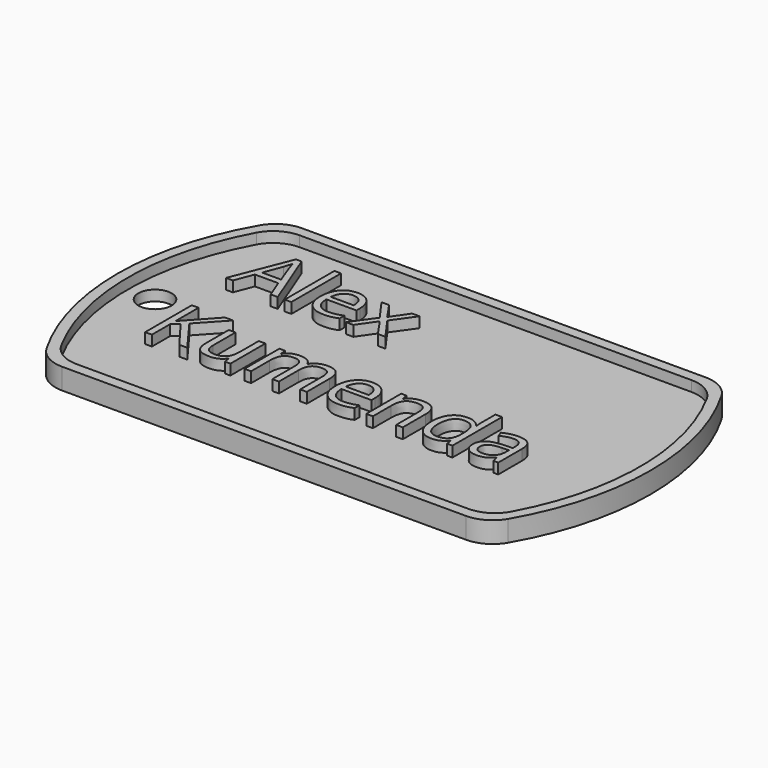
from build123d import *

# Parameters (mm, degrees)
F1_DEPTH     = 1
F3_DEPTH     = 1
F4_R         = 1.5875
F5_DEPTH     = 1
F6_TEXT_SIZE = 7.784575761
F7_DEPTH     = 1


# Not quite as in the source:
# - Text() gives the source's letters only with a copy of the font that has no kerning and outlines rounded to 1/6400 em; it was checked with that copy


with BuildPart() as f1:
    # F0 (on Top) → F1 (new body)
    with BuildSketch(Plane.XY):
        with BuildLine():
            ThreePointArc((-19.2474145991, 14.2875), (-20.8349145991, 13.862130657), (-21.9970452561, 12.7))
            ThreePointArc((-21.9970452561, 12.7), (-25.4, 0), (-21.9970452561, -12.7))
            ThreePointArc((-21.9970452561, -12.7), (-20.8349145991, -13.862130657), (-19.2474145991, -14.2875))
            Line((-19.2474145991, -14.2875), (19.2474145991, -14.2875))
            ThreePointArc((19.2474145991, -14.2875), (20.8349145991, -13.862130657), (21.9970452561, -12.7))
            ThreePointArc((21.9970452561, -12.7), (25.4, 0), (21.9970452561, 12.7))
            ThreePointArc((21.9970452561, 12.7), (20.8349145991, 13.862130657), (19.2474145991, 14.2875))
            Line((19.2474145991, 14.2875), (-19.2474145991, 14.2875))
        make_face()
    extrude(amount=F1_DEPTH)

    # F2 (on face) → F3 (join)
    with BuildSketch(Plane.XY.offset(1)):
        with BuildLine():
            Line((19.2474145991, 14.2875), (-19.2474145991, 14.2875))
            ThreePointArc((-19.2474145991, 14.2875), (-20.8349145991, 13.862130657), (-21.9970452561, 12.7))
            ThreePointArc((-21.9970452561, 12.7), (-25.4, 0), (-21.9970452561, -12.7))
            ThreePointArc((-21.9970452561, -12.7), (-20.8349145991, -13.862130657), (-19.2474145991, -14.2875))
            Line((-19.2474145991, -14.2875), (19.2474145991, -14.2875))
            ThreePointArc((19.2474145991, -14.2875), (20.8349145991, -13.862130657), (21.9970452561, -12.7))
            ThreePointArc((21.9970452561, -12.7), (25.4, 0), (21.9970452561, 12.7))
            ThreePointArc((21.9970452561, 12.7), (20.8349145991, 13.862130657), (19.2474145991, 14.2875))
        make_face()
        with BuildLine():
            ThreePointArc((-21.4526124879, 11.6252061249), (-20.2856017842, 12.8404540819), (-18.6611352482, 13.2875))
            Line((-18.6611352482, 13.2875), (18.6611352482, 13.2875))
            ThreePointArc((18.6611352482, 13.2875), (20.2856017842, 12.8404540819), (21.4526124879, 11.6252061249))
            ThreePointArc((21.4526124879, 11.6252061249), (24.4, 0), (21.4526124879, -11.6252061249))
            ThreePointArc((21.4526124879, -11.6252061249), (20.2856017842, -12.8404540819), (18.6611352482, -13.2875))
            Line((18.6611352482, -13.2875), (-18.6611352482, -13.2875))
            ThreePointArc((-18.6611352482, -13.2875), (-20.2856017842, -12.8404540819), (-21.4526124879, -11.6252061249))
            ThreePointArc((-21.4526124879, -11.6252061249), (-24.4, 0), (-21.4526124879, 11.6252061249))
        make_face(mode=Mode.SUBTRACT)
    extrude(amount=F3_DEPTH)

    # F4 (on face) → F5 (cut)
    with BuildSketch(Plane.XY.offset(1)):
        with Locations((-21.821282804, 0)):
            Circle(F4_R)
    extrude(amount=-F5_DEPTH, mode=Mode.SUBTRACT)

    # F6 (on face) → F7 (join)
    with BuildSketch(Plane.XY.offset(1)):
        with Locations((-18.6611352482, 4.5076054521)):
            Text('Alex', F6_TEXT_SIZE, font='Open Sans', text_align=(TextAlign.LEFT, TextAlign.BOTTOM))
        with Locations((-18.6611352482, -6.0794175828)):
            Text('Kumenda', F6_TEXT_SIZE, font='Open Sans', text_align=(TextAlign.LEFT, TextAlign.BOTTOM))
    extrude(amount=F7_DEPTH)


solid = f1.part
